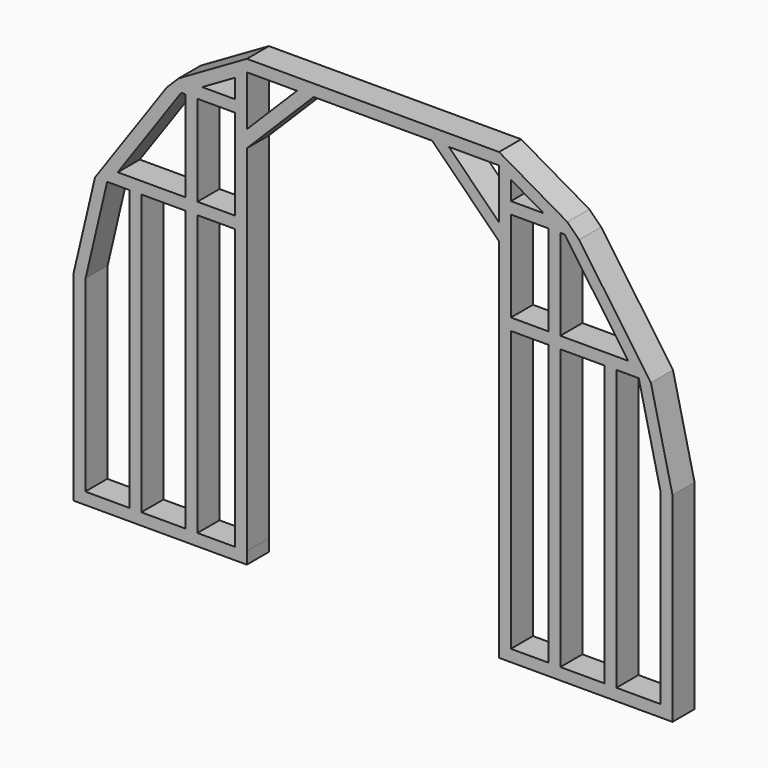
from build123d import *

# Parameters (mm, degrees)
F0_W     = 38.1
F0_H     = 605.4239357613
F0_H_2   = 901.7
F0_W_2   = 121.1758604333
F0_H_3   = 38.1
F1_DEPTH = 88.9


# Not quite as in the source:
# - a feature names something its author has since deleted; it is built from what else it names


with BuildPart() as f1:
    # F0 (on Front) → F1 (new body)
    with BuildSketch(Plane.XZ):
        Polygon((0, 38.1), (0, 0), (558.8, 0), (558.8, 38.1), (520.7027813, 38.1), (399.5269208667, 38.1), (361.4269208667, 38.1), (218.8134604333, 38.1), (180.7134604333, 38.1), (38.1, 38.1), align=None)
        with Locations((19.05, 340.8119678807)):
            Rectangle(F0_W, F0_H)
        Polygon((520.7027813, 38.1), (558.8, 38.1), (558.8027813, 38.1), (558.8027813, 939.8), (558.8027813, 1181.4738530943), (558.8027813, 1235.3553898208), (558.8027813, 1270), (520.7027813, 1270), (520.7027813, 977.9), (520.7027813, 939.8), align=None)
        Polygon((69.5237996219, 939.8), (0, 643.5239357613), (38.1, 643.5239357613), (39.1349278428, 643.5239357613), (108.6587274647, 939.8), align=None)
        with Locations((199.7634604333, 488.95)):
            Rectangle(F0_W, F0_H_2)
        Polygon((96.2017068277, 977.9), (69.5237996219, 939.8), (108.6587274647, 939.8), (180.7134604333, 939.8), (218.8134604333, 939.8), (361.4269208667, 939.8), (361.4269208667, 977.9), (142.7132186595, 977.9), align=None)
        Polygon((361.4269208667, 38.1), (399.5269208667, 38.1), (399.5269208667, 939.8), (399.5269208667, 977.9), (399.5269208667, 1270), (361.4269208667, 1270), (361.4269208667, 977.9), (361.4269208667, 939.8), align=None)
        with Locations((460.1148510833, 958.85)):
            Rectangle(F0_W_2, F0_H_3)
        Polygon((300.7323287388, 1270), (96.2017068277, 977.9), (142.7132186595, 977.9), (347.2438405706, 1270), align=None)
        Polygon((558.8027813, 1235.3553898208), (558.8027813, 1181.4738530943), (774.3289282057, 1397), (720.4473914792, 1397), align=None)
        Polygon((338.8323287388, 1308.1), (300.7323287388, 1270), (347.2438405706, 1270), (361.4269208667, 1270), (399.5269208667, 1270), (520.7027813, 1270), (558.8027813, 1270), (558.8027813, 1308.1), (520.7027813, 1308.1), (415.0323287388, 1308.1), (339.9874666667, 1308.1), align=None)
        Polygon((720.4473914792, 1397), (774.3289282057, 1397), (965.2027813, 1397), (965.2027813, 1435.1), (558.8027813, 1435.1), (558.8027813, 1397), align=None)
        Polygon((558.8027813, 1435.1), (338.8323287388, 1308.1), (339.9874666667, 1308.1), (415.0323287388, 1308.1), (520.7027813, 1369.1088642316), (558.8027813, 1391.1059094878), (558.8027813, 1397), align=None)
        Polygon((520.7027813, 1308.1), (558.8027813, 1308.1), (558.8027813, 1391.1059094878), (520.7027813, 1369.1088642316), align=None)
    extrude(amount=F1_DEPTH)

    # F2: F1 across face


with BuildPart() as f1_1:
    add(f1.part)
    add(f1.part.mirror(Plane(origin=(965.2027813, -44.45, 1416.05), x_dir=(0, 1, 0), z_dir=(1, 0, 0))))


solid = f1_1.part
